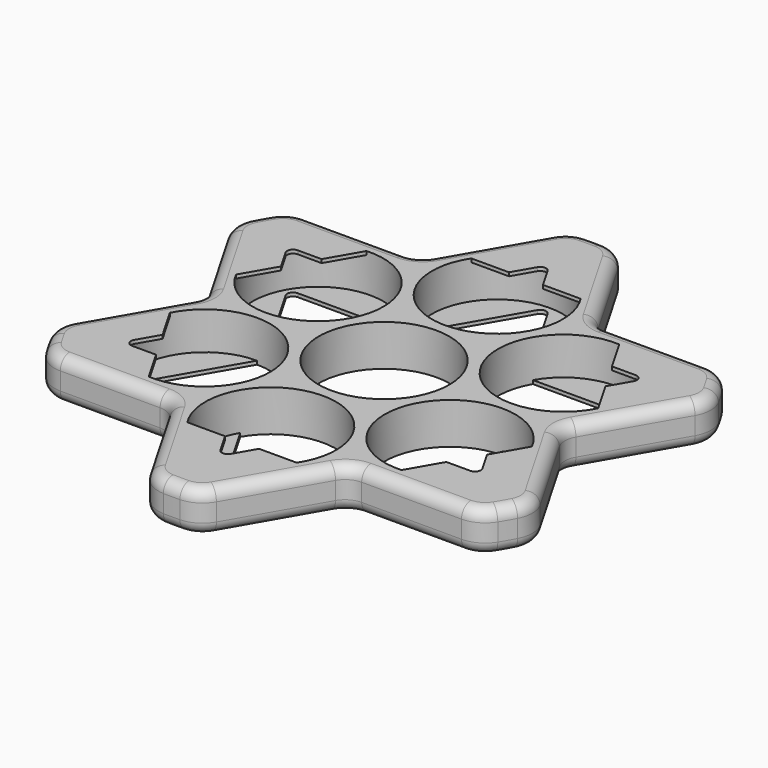
from build123d import *

# Parameters (mm, degrees)
F0_R            = 11.075
F1_DEPTH        = 7
F3_DEPTH        = 0.6
F3_COPIES_COUNT = 6
F5_DEPTH        = 0.6
F5_COPIES_COUNT = 6
F6_R            = 2


# Not quite as in the source:
# - a pattern or mirror of a feature is missing from the dataset's text; its kind, count and spacing are read off the source's solid


with BuildPart() as f1:
    # F0 (on Top) → F1 (new body)
    with BuildSketch(Plane.XY):
        with BuildLine():
            ThreePointArc((-38.247425235, -23.709375), (-36.4295958773, -25.4437455293), (-33.99771132, -26.075))
            Line((-33.99771132, -26.075), (-17.0751342113, -26.075))
            ThreePointArc((-17.0751342113, -26.075), (-15.3251342113, -26.5439110868), (-14.044045298, -27.825))
            Line((-14.044045298, -27.825), (-5.5827567437, -42.4803816737))
            ThreePointArc((-5.5827567437, -42.4803816737), (-3.8201320572, -44.270828244), (-1.4092084403, -44.9779293829))
            ThreePointArc((-1.4092084403, -44.9779293829), (0, -45), (1.4092084403, -44.9779293829))
            ThreePointArc((1.4092084403, -44.9779293829), (3.8201320572, -44.270828244), (5.5827567437, -42.4803816737))
            Line((5.5827567437, -42.4803816737), (14.044045298, -27.825))
            ThreePointArc((14.044045298, -27.825), (15.3251342113, -26.5439110868), (17.0751342113, -26.075))
            Line((17.0751342113, -26.075), (33.99771132, -26.075))
            ThreePointArc((33.99771132, -26.075), (36.4295958773, -25.4437455293), (38.247425235, -23.709375))
            ThreePointArc((38.247425235, -23.709375), (38.9711431703, -22.5), (39.6566336754, -21.2685543829))
            ThreePointArc((39.6566336754, -21.2685543829), (40.2497279345, -18.8270827147), (39.5804680637, -16.4053816737))
            Line((39.5804680637, -16.4053816737), (31.1191795093, -1.75))
            ThreePointArc((31.1191795093, -1.75), (30.6502684226, 0), (31.1191795093, 1.75))
            Line((31.1191795093, 1.75), (39.5804680637, 16.4053816737))
            ThreePointArc((39.5804680637, 16.4053816737), (40.2497279345, 18.8270827147), (39.6566336754, 21.2685543829))
            ThreePointArc((39.6566336754, 21.2685543829), (38.9711431703, 22.5), (38.247425235, 23.709375))
            ThreePointArc((38.247425235, 23.709375), (36.4295958773, 25.4437455293), (33.99771132, 26.075))
            Line((33.99771132, 26.075), (17.0751342113, 26.075))
            ThreePointArc((17.0751342113, 26.075), (15.3251342113, 26.5439110868), (14.044045298, 27.825))
            Line((14.044045298, 27.825), (5.5827567437, 42.4803816737))
            ThreePointArc((5.5827567437, 42.4803816737), (3.8201320572, 44.270828244), (1.4092084403, 44.9779293829))
            ThreePointArc((1.4092084403, 44.9779293829), (0, 45), (-1.4092084403, 44.9779293829))
            ThreePointArc((-1.4092084403, 44.9779293829), (-3.8201320572, 44.270828244), (-5.5827567437, 42.4803816737))
            Line((-5.5827567437, 42.4803816737), (-14.044045298, 27.825))
            ThreePointArc((-14.044045298, 27.825), (-15.3251342113, 26.5439110868), (-17.0751342113, 26.075))
            Line((-17.0751342113, 26.075), (-33.99771132, 26.075))
            ThreePointArc((-33.99771132, 26.075), (-36.4295958773, 25.4437455293), (-38.247425235, 23.709375))
            ThreePointArc((-38.247425235, 23.709375), (-38.9711431703, 22.5), (-39.6566336754, 21.2685543829))
            ThreePointArc((-39.6566336754, 21.2685543829), (-40.2497279345, 18.8270827147), (-39.5804680637, 16.4053816737))
            Line((-39.5804680637, 16.4053816737), (-31.1191795093, 1.75))
            ThreePointArc((-31.1191795093, 1.75), (-30.6502684226, 0), (-31.1191795093, -1.75))
            Line((-31.1191795093, -1.75), (-39.5804680637, -16.4053816737))
            ThreePointArc((-39.5804680637, -16.4053816737), (-40.2497279345, -18.8270827147), (-39.6566336754, -21.2685543829))
            ThreePointArc((-39.6566336754, -21.2685543829), (-38.9711431703, -22.5), (-38.247425235, -23.709375))
        make_face()
        with Locations((-20.7846096908, -12)):
            Circle(F0_R, mode=Mode.SUBTRACT)
        with Locations((0, -24)):
            Circle(F0_R, mode=Mode.SUBTRACT)
        with Locations((20.7846096908, -12)):
            Circle(F0_R, mode=Mode.SUBTRACT)
        with Locations((-20.7846096908, 12)):
            Circle(F0_R, mode=Mode.SUBTRACT)
        Circle(F0_R, mode=Mode.SUBTRACT)
        with Locations((20.7846096908, 12)):
            Circle(F0_R, mode=Mode.SUBTRACT)
        with Locations((0, 24)):
            Circle(F0_R, mode=Mode.SUBTRACT)
    extrude(amount=F1_DEPTH)

    # F2 (on face) → F3 (join)
    with BuildSketch(Plane(origin=(0, 0, 0), x_dir=(1, 0, 0), z_dir=(0, 0, -1))):
        with BuildLine():
            ThreePointArc((-9.5912313469, -18.4625), (0, -35.075), (9.5912313469, -18.4625))
            Line((9.5912313469, -18.4625), (0.8660254038, -33.575))
            ThreePointArc((0.8660254038, -33.575), (0, -34.075), (-0.8660254038, -33.575))
            Line((-0.8660254038, -33.575), (-9.5912313469, -18.4625))
        make_face()
    f3 = extrude(amount=-F3_DEPTH)

    # F3_copies: F3 ×6 about axis
    f3_copies_axis = Axis((0, 0, 0), (0, 0, 1))
    for i in range(1, F3_COPIES_COUNT):
        add(f3.rotate(f3_copies_axis, i * 360 / F3_COPIES_COUNT))

    # F4 (on face) → F5 (join)
    with BuildSketch(Plane.XY.offset(7)):
        with BuildLine():
            Line((-9.2601295887, 30.075), (-2.8867513459, 30.075))
            Line((-2.8867513459, 30.075), (-0.8660254038, 33.575))
            ThreePointArc((-0.8660254038, 33.575), (0, 34.075), (0.8660254038, 33.575))
            Line((0.8660254038, 33.575), (2.8867513459, 30.075))
            Line((2.8867513459, 30.075), (9.2601295887, 30.075))
            ThreePointArc((9.2601295887, 30.075), (0, 35.075), (-9.2601295887, 30.075))
        make_face()
    f5 = extrude(amount=-F5_DEPTH)

    # F5_copies: F5 ×6 about axis
    f5_copies_axis = Axis((0, 0, 0), (0, 0, 1))
    for i in range(1, F5_COPIES_COUNT):
        add(f5.rotate(f5_copies_axis, i * 360 / F5_COPIES_COUNT))

    # F6
    f6_edges = [f1.edges().sort_by_distance(p)[0] for p in [
        (-25.536423, -26.075, 7),
        (-25.536423, -26.075, 0),
        (38.971143, -22.5, 0),
        (38.971143, -22.5, 7),
        (36.429596, -25.443746, 0),
        (36.429596, -25.443746, 7),
        (40.249728, -18.827083, 0),
        (40.249728, -18.827083, 7),
        (35.349824, -9.077691, 0),
        (30.650268, 0, 0),
        (35.349824, 9.077691, 0),
        (40.249728, 18.827083, 0),
        (38.971143, 22.5, 0),
        (36.429596, 25.443746, 0),
        (25.536423, 26.075, 0),
        (15.325134, 26.543911, 0),
        (9.813401, 35.152691, 0),
        (3.820132, 44.270828, 0),
        (0, 45, 0),
        (-3.820132, 44.270828, 0),
        (-9.813401, 35.152691, 0),
        (-15.325134, 26.543911, 0),
        (-25.536423, 26.075, 0),
        (-36.429596, 25.443746, 0),
        (-38.971143, 22.5, 0),
        (-40.249728, 18.827083, 0),
        (-35.349824, 9.077691, 0),
        (-30.650268, 0, 0),
        (-35.349824, -9.077691, 0),
        (-40.249728, -18.827083, 0),
        (-38.971143, -22.5, 0),
        (-36.429596, -25.443746, 0),
        (-15.325134, -26.543911, 0),
        (-9.813401, -35.152691, 0),
        (-3.820132, -44.270828, 0),
        (0, -45, 0),
        (3.820132, -44.270828, 0),
        (9.813401, -35.152691, 0),
        (15.325134, -26.543911, 0),
        (25.536423, -26.075, 0),
        (35.349824, -9.077691, 7),
        (30.650268, 0, 7),
        (35.349824, 9.077691, 7),
        (40.249728, 18.827083, 7),
        (38.971143, 22.5, 7),
        (36.429596, 25.443746, 7),
        (25.536423, 26.075, 7),
        (15.325134, 26.543911, 7),
        (9.813401, 35.152691, 7),
        (3.820132, 44.270828, 7),
        (0, 45, 7),
        (-3.820132, 44.270828, 7),
        (-9.813401, 35.152691, 7),
        (-15.325134, 26.543911, 7),
        (-25.536423, 26.075, 7),
        (-36.429596, 25.443746, 7),
        (-38.971143, 22.5, 7),
        (-40.249728, 18.827083, 7),
        (-35.349824, 9.077691, 7),
        (-30.650268, 0, 7),
        (-35.349824, -9.077691, 7),
        (-40.249728, -18.827083, 7),
        (-38.971143, -22.5, 7),
        (-36.429596, -25.443746, 7),
        (-15.325134, -26.543911, 7),
        (-9.813401, -35.152691, 7),
        (-3.820132, -44.270828, 7),
        (0, -45, 7),
        (3.820132, -44.270828, 7),
        (9.813401, -35.152691, 7),
        (15.325134, -26.543911, 7),
        (25.536423, -26.075, 7),
    ]]
    fillet(f6_edges, radius=F6_R)


solid = f1.part
